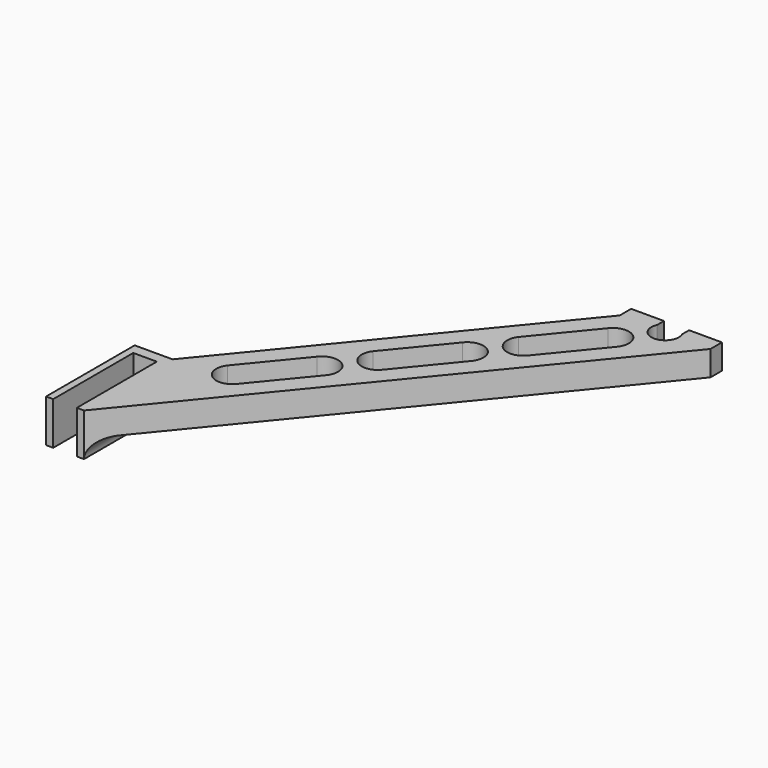
from build123d import *

# Parameters (mm, degrees)
F1_DEPTH = 12
F2_DEPTH = 25
F3_DEPTH = 5
F4_R     = 4.99999


# Not quite as in the source:
# - a fillet or chamfer is up to 0.001 mm smaller than in the source, because OpenCascade refuses the exact size


with BuildPart() as f1:
    # F0 (on Top) → F1 (new body)
    with BuildSketch(Plane.XY):
        with BuildLine():
            Line((-45.8308390021, -20.6945241443), (-45.8308390021, -51.6945241443))
            Line((-45.8308390021, -51.6945241443), (42.9120542584, 56.586124615))
            Line((42.9120542584, 56.586124615), (42.9120542584, 60.586124615))
            Line((42.9120542584, 60.586124615), (33.7120542584, 60.586124615))
            Line((33.7120542584, 60.586124615), (33.7120542584, 58.1829414275))
            ThreePointArc((33.7120542584, 58.1829414275), (30.2088163179, 52.736124615), (26.7055783775, 58.1829414275))
            Line((26.7055783775, 58.1829414275), (26.7055783775, 60.586124615))
            Line((26.7055783775, 60.586124615), (17.5055783775, 60.586124615))
            Line((17.5055783775, 60.586124615), (17.5055783775, 56.586124615))
            Line((17.5055783775, 56.586124615), (-45.8308390021, -20.6945241443))
        make_face()
        with BuildLine():
            ThreePointArc((-27.6003750582, -21.0494093167), (-33.898601194, -21.7061227773), (-34.6189265027, -15.4148545048))
            Line((-34.6189265027, -15.4148545048), (-21.9413703226, 0.0538096037))
            ThreePointArc((-21.9413703226, 0.0538096037), (-15.5862024886, 0.7814511592), (-14.9228188782, -5.5807452082))
            Line((-14.9228188782, -5.5807452082), (-27.6003750582, -21.0494093167))
        make_face(mode=Mode.SUBTRACT)
        with BuildLine():
            ThreePointArc((-6.9814485555, 4.0654451881), (-13.2796746913, 3.4087317275), (-14, 9.7))
            Line((-14, 9.7), (-1.3224438199, 25.1686641085))
            ThreePointArc((-1.3224438199, 25.1686641085), (5.0327240141, 25.896305664), (5.6961076246, 19.5341092966))
            Line((5.6961076246, 19.5341092966), (-6.9814485555, 4.0654451881))
        make_face(mode=Mode.SUBTRACT)
        with BuildLine():
            ThreePointArc((13.6374779472, 29.1802996929), (7.3392518114, 28.5235862323), (6.6189265027, 34.8148545048))
            Line((6.6189265027, 34.8148545048), (19.2964826828, 50.2835186133))
            ThreePointArc((19.2964826828, 50.2835186133), (25.6516505168, 51.0111601688), (26.3150341273, 44.6489638014))
            Line((26.3150341273, 44.6489638014), (13.6374779472, 29.1802996929))
        make_face(mode=Mode.SUBTRACT)
        Polygon((-54.4308390021, -51.6945241443), (-54.4308390021, -23.6945241443), (-47.8308390021, -23.6945241443), (-47.8308390021, -51.6945241443), (-45.8308390021, -51.6945241443), (-45.8308390021, -20.6945241443), (-56.4308390021, -20.6945241443), (-56.4308390021, -51.6945241443), align=None)
    extrude(amount=F1_DEPTH)

    # F0 (on Top) → F2 (cut)
    with BuildSketch(Plane.XY):
        with BuildLine():
            Line((-21.9413703226, 0.0538096037), (-34.6189265027, -15.4148545048))
            ThreePointArc((-34.6189265027, -15.4148545048), (-33.898601194, -21.7061227773), (-27.6003750582, -21.0494093167))
            Line((-27.6003750582, -21.0494093167), (-14.9228188782, -5.5807452082))
            ThreePointArc((-14.9228188782, -5.5807452082), (-15.5862024886, 0.7814511592), (-21.9413703226, 0.0538096037))
        make_face()
        with BuildLine():
            Line((-1.3224438199, 25.1686641085), (-14, 9.7))
            ThreePointArc((-14, 9.7), (-13.2796746913, 3.4087317275), (-6.9814485555, 4.0654451881))
            Line((-6.9814485555, 4.0654451881), (5.6961076246, 19.5341092966))
            ThreePointArc((5.6961076246, 19.5341092966), (5.0327240141, 25.896305664), (-1.3224438199, 25.1686641085))
        make_face()
        with BuildLine():
            Line((19.2964826828, 50.2835186133), (6.6189265027, 34.8148545048))
            ThreePointArc((6.6189265027, 34.8148545048), (7.3392518114, 28.5235862323), (13.6374779472, 29.1802996929))
            Line((13.6374779472, 29.1802996929), (26.3150341273, 44.6489638014))
            ThreePointArc((26.3150341273, 44.6489638014), (25.6516505168, 51.0111601688), (19.2964826828, 50.2835186133))
        make_face()
    extrude(amount=-F2_DEPTH, mode=Mode.SUBTRACT)

    # F0 (on Top) → F3 (cut)
    with BuildSketch(Plane.XY):
        with BuildLine():
            Line((-45.8308390021, -20.6945241443), (-45.8308390021, -51.6945241443))
            Line((-45.8308390021, -51.6945241443), (42.9120542584, 56.586124615))
            Line((42.9120542584, 56.586124615), (42.9120542584, 60.586124615))
            Line((42.9120542584, 60.586124615), (33.7120542584, 60.586124615))
            Line((33.7120542584, 60.586124615), (33.7120542584, 58.1829414275))
            ThreePointArc((33.7120542584, 58.1829414275), (30.2088163179, 52.736124615), (26.7055783775, 58.1829414275))
            Line((26.7055783775, 58.1829414275), (26.7055783775, 60.586124615))
            Line((26.7055783775, 60.586124615), (17.5055783775, 60.586124615))
            Line((17.5055783775, 60.586124615), (17.5055783775, 56.586124615))
            Line((17.5055783775, 56.586124615), (-45.8308390021, -20.6945241443))
        make_face()
        with BuildLine():
            ThreePointArc((-27.6003750582, -21.0494093167), (-33.898601194, -21.7061227773), (-34.6189265027, -15.4148545048))
            Line((-34.6189265027, -15.4148545048), (-21.9413703226, 0.0538096037))
            ThreePointArc((-21.9413703226, 0.0538096037), (-15.5862024886, 0.7814511592), (-14.9228188782, -5.5807452082))
            Line((-14.9228188782, -5.5807452082), (-27.6003750582, -21.0494093167))
        make_face(mode=Mode.SUBTRACT)
        with BuildLine():
            ThreePointArc((-6.9814485555, 4.0654451881), (-13.2796746913, 3.4087317275), (-14, 9.7))
            Line((-14, 9.7), (-1.3224438199, 25.1686641085))
            ThreePointArc((-1.3224438199, 25.1686641085), (5.0327240141, 25.896305664), (5.6961076246, 19.5341092966))
            Line((5.6961076246, 19.5341092966), (-6.9814485555, 4.0654451881))
        make_face(mode=Mode.SUBTRACT)
        with BuildLine():
            ThreePointArc((13.6374779472, 29.1802996929), (7.3392518114, 28.5235862323), (6.6189265027, 34.8148545048))
            Line((6.6189265027, 34.8148545048), (19.2964826828, 50.2835186133))
            ThreePointArc((19.2964826828, 50.2835186133), (25.6516505168, 51.0111601688), (26.3150341273, 44.6489638014))
            Line((26.3150341273, 44.6489638014), (13.6374779472, 29.1802996929))
        make_face(mode=Mode.SUBTRACT)
    extrude(amount=F3_DEPTH, mode=Mode.SUBTRACT)

    # F4 (radius 5 in the source; OpenCascade refuses exactly that, so slightly less here)
    f4_edges = [f1.edges().sort_by_distance(p)[0] for p in [
        (-45.830839, -36.194524, 5),
    ]]
    fillet(f4_edges, radius=F4_R)


solid = f1.part
